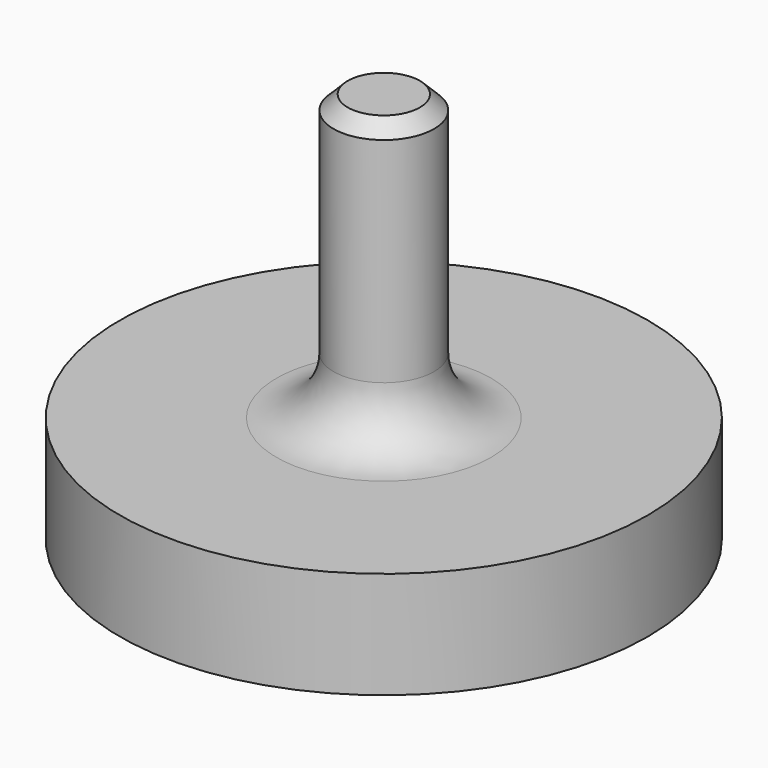
from build123d import *

# Parameters (mm, degrees)
F2_SIZE = 20


with BuildPart() as f1:
    # F0 (on Front) → F1 (revolve)
    with BuildSketch(Plane.XZ):
        with BuildLine():
            Line((0, 350.3882980986), (0, -350))
            Line((0, -350), (370.6526133659, -199.6117019014))
            Line((370.6526133659, -199.6117019014), (370.6526133659, -49.6117019014))
            Line((370.6526133659, -49.6117019014), (150.6526133659, -49.6117019014))
            ThreePointArc((150.6526133659, -49.6117019014), (94.084070871, -26.1802443963), (70.6526133659, 30.3882980986))
            Line((70.6526133659, 30.3882980986), (70.6526133659, 350.3882980986))
            Line((70.6526133659, 350.3882980986), (0, 350.3882980986))
        make_face()
    revolve(axis=Axis((0, 0, 0.1941490493), (0, 0, -1)))

    # F2
    f2_edges = [f1.edges().sort_by_distance(p)[0] for p in [
        (-70.652613, 0, 350.388298),
    ]]
    chamfer(f2_edges, length=F2_SIZE)


solid = f1.part
